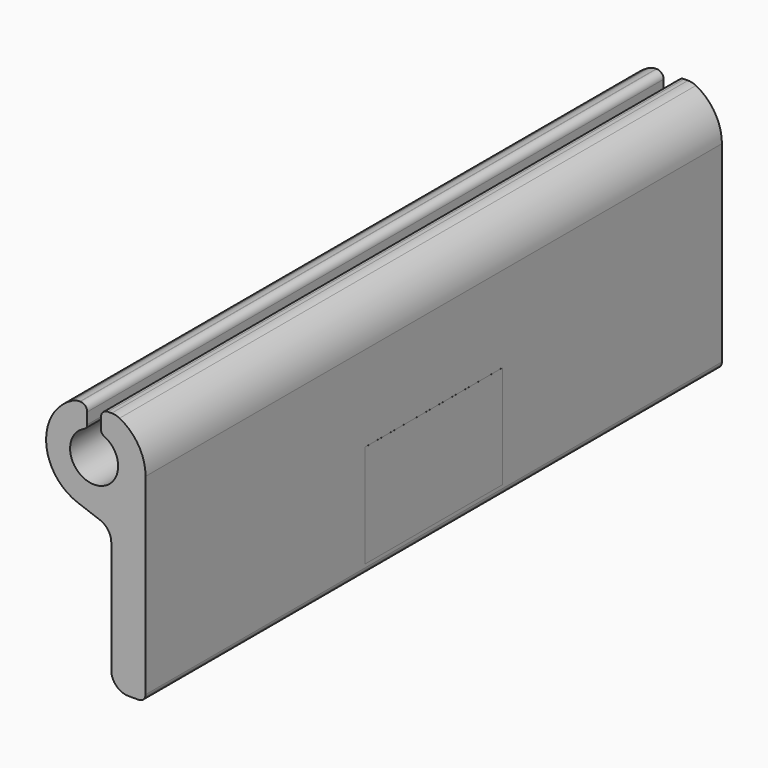
from build123d import *

# Parameters (mm, degrees)
F1_DEPTH = 105
F2_R     = 12
F3_DEPTH = 0.05
F4_W     = 50
F4_H     = 30
F5_DEPTH = 0.01


# Not quite as in the source:
# - ends of sketch curves that miss each other by under 0.0002 mm in the source are joined


with BuildPart() as f1:
    # F0 (on Front) → F1 (new body, symmetric)
    with BuildSketch(Plane.XZ):
        with BuildLine():
            Line((4.4999999997, -23.5), (4.4999999997, -30.5))
            ThreePointArc((4.4999999997, -30.5), (5.9644660938, -34.0355339059), (9.4999999997, -35.5))
            Line((9.4999999997, -35.5), (12.5, -35.5))
            ThreePointArc((12.5, -35.5), (13.9142133287, -34.9142135624), (14.4999997663, -33.5))
            Line((14.4999997663, -33.5), (14.4999997663, 22.4999994828))
            ThreePointArc((14.4999997663, 22.4999994828), (12.4539129776, 29.7872458033), (6.9137199183, 34.9444437777))
            ThreePointArc((6.9137199183, 34.9444437777), (5.8016169865, 35.3591259101), (4.6231056877, 35.4999993303))
            Line((4.6231056877, 35.4999993303), (3.4999997663, 35.4999993303))
            ThreePointArc((3.4999997663, 35.4999993303), (2.0857862039, 34.9142128927), (1.4999997663, 33.4999993303))
            Line((1.4999997663, 33.4999993303), (1.4999997663, 30.2459664828))
            ThreePointArc((1.4999997663, 30.2459664828), (1.7397477835, 29.4324771221), (2.3823530195, 28.8790310431))
            ThreePointArc((2.3823530195, 28.8790310431), (-0.5000000985, 15.4999997293), (-3.3823532363, 28.8790310342))
            ThreePointArc((-3.3823532363, 28.8790310342), (-2.7397478169, 29.4324771961), (-2.4999997997, 30.2459665567))
            Line((-2.4999997997, 30.2459665567), (-2.4999997997, 33.5))
            ThreePointArc((-2.4999997997, 33.5), (-3.0857862373, 34.9142132361), (-4.4999997997, 35.4999996738))
            Line((-4.4999997997, 35.4999996738), (-4.6231058319, 35.4999996738))
            ThreePointArc((-4.6231058319, 35.4999996738), (-5.8016171306, 35.3591262536), (-6.9137200625, 34.9444441212))
            ThreePointArc((-6.9137200625, 34.9444441212), (-14.4718653147, 21.6128794539), (-5.288282, 9.344303))
            Line((-5.288282, 9.344303), (1.210101, 6.979085))
            ThreePointArc((1.210101, 6.979085), (3.5957603078, 5.1485040574), (4.4999999997, 2.2806219993))
            Line((4.4999999997, 2.2806219993), (4.4999999997, 0.5))
            Line((4.4999999997, 0.5), (4.4999999997, -23.5))
        make_face()
    extrude(amount=F1_DEPTH, both=True)

    # F2 (on face) → F3 (join)
    with BuildSketch(Plane(origin=(4.4999999997, 0, 0), x_dir=(0, -1, 0), z_dir=(-1, 0, 0))):
        with Locations((0, -11.5)):
            Circle(F2_R)
    extrude(amount=F3_DEPTH)

    # F4 (on face) → F5 (join)
    with BuildSketch(Plane.YZ.offset(14.4999997663)):
        with Locations((0, -17.5000005172)):
            Rectangle(F4_W, F4_H)
    extrude(amount=F5_DEPTH)


solid = f1.part
